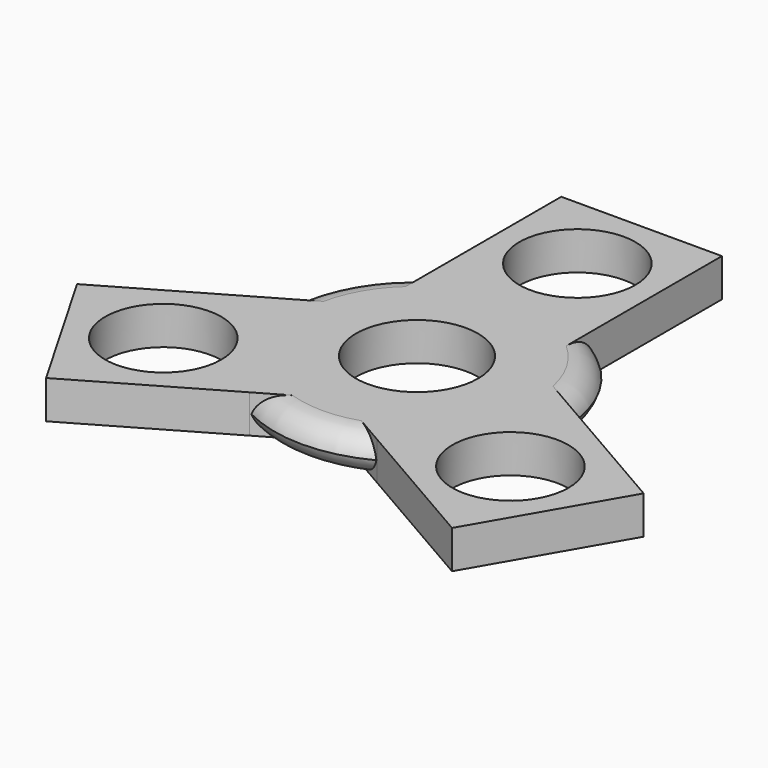
from build123d import *

# Parameters (mm, degrees)
F0_W         = 29.492739588
F0_H         = 29.492739588
F0_R         = 10.6622653611
F0_R_2       = 13.2
F0_R_3       = 11.2
F1_DEPTH     = 7
F2_T4_ANGLE  = 112.5181364767
F2_T10_ANGLE = 112.5181364767
F2_T16_ANGLE = 112.5181364767
F2_T22_ANGLE = 112.5181364767
F2_T28_ANGLE = 112.5181364767
F2_T34_ANGLE = 112.5181364767


# Not quite as in the source:
# - a fillet or chamfer that OpenCascade refuses, or shapes differently, is made with other operations: its cross-section is extruded or revolved along the edge and cut away or added


with BuildPart() as f1:
    # F0 (on Top) → F1 (new body)
    with BuildSketch(Plane.XY):
        with Locations((0, 36.7929209024)):
            Rectangle(F0_W, F0_H)
        with Locations((0, 36.7929209024)):
            Circle(F0_R, mode=Mode.SUBTRACT)
        with BuildLine():
            Line((14.746369794, 22.0465511084), (-14.746369794, 22.0465511084))
            ThreePointArc((-14.746369794, 22.0465511084), (-23.115726428, 13.3458708757), (-26.4660582227, 1.747455301))
            Line((-26.4660582227, 1.747455301), (-11.7196884287, -23.7940064094))
            ThreePointArc((-11.7196884287, -23.7940064094), (0, -26.6917417515), (11.7196884287, -23.7940064094))
            Line((11.7196884287, -23.7940064094), (26.4660582227, 1.747455301))
            ThreePointArc((26.4660582227, 1.747455301), (23.115726428, 13.3458708757), (14.746369794, 22.0465511084))
        make_face()
        Circle(F0_R_2, mode=Mode.SUBTRACT)
        Polygon((52.0075199331, -12.998914493), (26.4660582227, 1.747455301), (11.7196884287, -23.7940064094), (37.2611501391, -38.5403762034), align=None)
        with Locations((31.8636041809, -18.3964604512)):
            Circle(F0_R, mode=Mode.SUBTRACT)
        Polygon((-11.7196884287, -23.7940064094), (-26.4660582227, 1.747455301), (-52.0075199331, -12.998914493), (-37.2611501391, -38.5403762034), align=None)
        with Locations((-31.8636041809, -18.3964604512)):
            Circle(F0_R, mode=Mode.SUBTRACT)
        Circle(F0_R_2)
        Circle(F0_R_3, mode=Mode.SUBTRACT)
    extrude(amount=F1_DEPTH)

    # F2: fillet of radius 5 on 6 edges, made by hand


with BuildPart() as f2_tool2:
    # F2_s3 → F2_t4 (revolve)
    with BuildSketch(Plane(origin=(-1.2804779727, -0.0837234298, 0), x_dir=(0, 0, 1), z_dir=(0.9978692621, 0.0652451967, 0))):
        with BuildLine():
            ThreePointArc((2, -26.0057199962), (5.5355339059, -24.5412539021), (7, -21.0057199962))
            Line((7, -21.0057199962), (7, -26.0057199962))
            Line((7, -26.0057199962), (2, -26.0057199962))
        make_face()
    revolve(axis=Axis((-1.336401015, 0.7715714858, 7), (0, 0, 1)), revolution_arc=F2_T4_ANGLE)

    split(bisect_by=Plane.YZ.offset(-14.746369794), keep=Keep.BOTTOM)

    split(bisect_by=Plane(origin=(-7.373184897, 12.7707308552, 0), x_dir=(0, 0, 1), z_dir=(-0.5, 0.8660254038, 0)), keep=Keep.TOP)


with BuildPart() as f1_1:
    add(f1.part)

    # F2_t1: cut F2_tool2
    add(f2_tool2.part, mode=Mode.SUBTRACT)


with BuildPart() as f2_tool8:
    # F2_s9 → F2_t10 (revolve)
    with BuildSketch(Plane(origin=(0.5677323692, 1.1507881683, 0), x_dir=(0, 0, 1), z_dir=(-0.4424306333, -0.896802729, 0))):
        with BuildLine():
            ThreePointArc((2, -26.0057199962), (5.5355339059, -24.5412539021), (7, -21.0057199962))
            Line((7, -21.0057199962), (7, -26.0057199962))
            Line((7, -26.0057199962), (2, -26.0057199962))
        make_face()
    revolve(axis=Axis((1.336401015, 0.7715714858, 7), (0, 0, 1)), revolution_arc=F2_T10_ANGLE)

    split(bisect_by=Plane(origin=(7.373184897, 12.7707308552, 0), x_dir=(0, 0, 1), z_dir=(0.5, 0.8660254038, 0)), keep=Keep.TOP)

    split(bisect_by=Plane.YZ.offset(14.746369794), keep=Keep.TOP)


with BuildPart() as f1_2:
    add(f1_1.part)

    # F2_t7: cut F2_tool8
    add(f2_tool8.part, mode=Mode.SUBTRACT)


with BuildPart() as f2_tool14:
    # F2_s15 → F2_t16 (revolve)
    with BuildSketch(Plane(origin=(0.7127456035, -1.0670647384, 0), x_dir=(0, 0, 1), z_dir=(-0.5554386289, 0.8315575323, 0))):
        with BuildLine():
            ThreePointArc((2, -26.0057199962), (5.5355339059, -24.5412539021), (7, -21.0057199962))
            Line((7, -21.0057199962), (7, -26.0057199962))
            Line((7, -26.0057199962), (2, -26.0057199962))
        make_face()
    revolve(axis=Axis((0, -1.5431429715, 7), (0, 0, 1)), revolution_arc=F2_T16_ANGLE)

    split(bisect_by=Plane(origin=(7.373184897, -12.7707308552, 0), x_dir=(0, 0, 1), z_dir=(0.5, -0.8660254038, 0)), keep=Keep.TOP)

    split(bisect_by=Plane(origin=(-7.373184897, -12.7707308552, 0), x_dir=(0, 0, 1), z_dir=(-0.5, -0.8660254038, 0)), keep=Keep.TOP)


with BuildPart() as f1_3:
    add(f1_2.part)

    # F2_t13: cut F2_tool14
    add(f2_tool14.part, mode=Mode.SUBTRACT)


with BuildPart() as f2_tool20:
    # F2_s21 → F2_t22 (revolve)
    with BuildSketch(Plane(origin=(0.5677323692, 1.1507881683, 0), x_dir=(0, 0, 1), z_dir=(-0.4424306333, -0.896802729, 0))):
        with BuildLine():
            ThreePointArc((5, -26.0057199962), (1.4644660941, -24.5412539021), (0, -21.0057199962))
            Line((0, -21.0057199962), (0, -26.0057199962))
            Line((0, -26.0057199962), (5, -26.0057199962))
        make_face()
    revolve(axis=Axis((1.336401015, 0.7715714858, 0), (0, 0, 1)), revolution_arc=F2_T22_ANGLE)

    split(bisect_by=Plane(origin=(7.373184897, 12.7707308552, 0), x_dir=(0, 0, 1), z_dir=(0.5, 0.8660254038, 0)), keep=Keep.TOP)

    split(bisect_by=Plane.YZ.offset(14.746369794), keep=Keep.TOP)


with BuildPart() as f1_4:
    add(f1_3.part)

    # F2_t19: cut F2_tool20
    add(f2_tool20.part, mode=Mode.SUBTRACT)


with BuildPart() as f2_tool26:
    # F2_s27 → F2_t28 (revolve)
    with BuildSketch(Plane(origin=(0.7127456035, -1.0670647384, 0), x_dir=(0, 0, 1), z_dir=(-0.5554386289, 0.8315575323, 0))):
        with BuildLine():
            ThreePointArc((5, -26.0057199962), (1.4644660941, -24.5412539021), (0, -21.0057199962))
            Line((0, -21.0057199962), (0, -26.0057199962))
            Line((0, -26.0057199962), (5, -26.0057199962))
        make_face()
    revolve(axis=Axis((0, -1.5431429715, 0), (0, 0, 1)), revolution_arc=F2_T28_ANGLE)

    split(bisect_by=Plane(origin=(7.373184897, -12.7707308552, 0), x_dir=(0, 0, 1), z_dir=(0.5, -0.8660254038, 0)), keep=Keep.TOP)

    split(bisect_by=Plane(origin=(-7.373184897, -12.7707308552, 0), x_dir=(0, 0, 1), z_dir=(-0.5, -0.8660254038, 0)), keep=Keep.TOP)


with BuildPart() as f1_5:
    add(f1_4.part)

    # F2_t25: cut F2_tool26
    add(f2_tool26.part, mode=Mode.SUBTRACT)


with BuildPart() as f2_tool32:
    # F2_s33 → F2_t34 (revolve)
    with BuildSketch(Plane(origin=(-1.2804779727, -0.0837234298, 0), x_dir=(0, 0, 1), z_dir=(0.9978692621, 0.0652451967, 0))):
        with BuildLine():
            ThreePointArc((5, -26.0057199962), (1.4644660941, -24.5412539021), (0, -21.0057199962))
            Line((0, -21.0057199962), (0, -26.0057199962))
            Line((0, -26.0057199962), (5, -26.0057199962))
        make_face()
    revolve(axis=Axis((-1.336401015, 0.7715714858, 0), (0, 0, 1)), revolution_arc=F2_T34_ANGLE)

    split(bisect_by=Plane.YZ.offset(-14.746369794), keep=Keep.BOTTOM)

    split(bisect_by=Plane(origin=(-7.373184897, 12.7707308552, 0), x_dir=(0, 0, 1), z_dir=(-0.5, 0.8660254038, 0)), keep=Keep.TOP)


with BuildPart() as f1_6:
    add(f1_5.part)

    # F2_t31: cut F2_tool32
    add(f2_tool32.part, mode=Mode.SUBTRACT)


solid = f1_6.part
